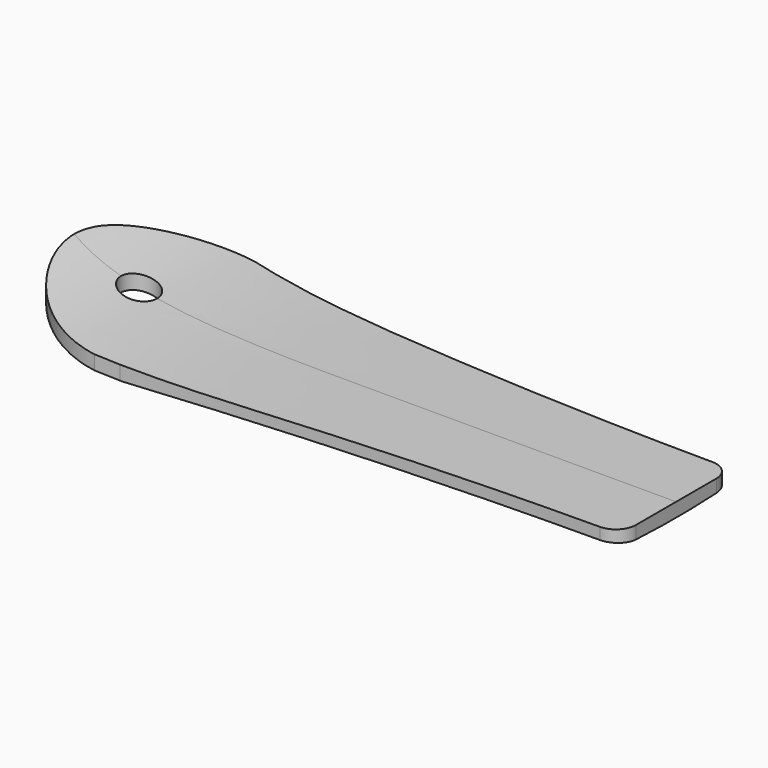
from build123d import *

# Parameters (mm, degrees)
F2_DEPTH = 50
F0_R     = 9
F3_DEPTH = 41
F5_DEPTH = 150


# Not quite as in the source:
# - the dataset's text gives a spline's control points without its knots; the knots are read off the source's solid


with BuildPart() as f2:
    # F1 (on Front) → F2 (new body, symmetric)
    with BuildSketch(Plane.XZ):
        with BuildLine():
            ThreePointArc((-149.9588993892, 26.9134754342), (-154.8613095864, 26.2305586605), (-154.1783928127, 21.3281484633))
            add(Edge.make_bspline(
                [(-154.1783928127, 21.3281484633), (-125.9464059615, 0), (-3.9595449586, 0), (130.4603123693, 0), (151.5675187111, 0)],
                knots=[0, 0, 0, 0, 0.5033195654, 1, 1, 1, 1], degree=3))
            ThreePointArc((151.5675187111, 0), (155.0675187869, 3.5000000758), (151.5675187111, 7.0000001516))
            add(Edge.make_bspline(
                [(-149.9588993892, 26.9134754342), (-148.4478574546, 25.7719430693), (-145.1555512603, 23.5934371829), (-137.5039021405, 19.6641031988), (-126.0184700843, 15.5798750303), (-109.5578013858, 11.9753296087), (-90.8479253185, 9.5246754809), (-70.2937339258, 8.030291433), (-48.2800158692, 7.2686571064), (-29.0264464578, 7.0487772943), (-13.2581336189, 7.0012099028), (-1.291744917, 6.9996863373), (10.7653391732, 7.0000823662), (26.8484793874, 6.9999526881), (46.7909432723, 7.0000162503), (69.87873725, 6.9999959326), (98.7623960141, 7.0000025942), (129.847702251, 6.9999992634), (146.255449604, 7.0000001516), (151.5675187111, 7.0000001516)],
                knots=[0, 0, 0, 0, 0.03125, 0.0625, 0.125, 0.1875, 0.25, 0.3125, 0.375, 0.4375, 0.46875, 0.5, 0.53125, 0.5625, 0.625, 0.6875, 0.75, 0.875, 1, 1, 1, 1], degree=3))
        make_face()
    extrude(amount=F2_DEPTH, both=True)

    # F0 (on Top) → F3 (intersect)
    with BuildSketch(Plane.XY):
        with BuildLine():
            ThreePointArc((-150, 0), (-135.3553390593, -35.3553390593), (-100, -50))
            ThreePointArc((-100, -50), (-94.2011170994, -49.3098342645), (-88.4003291499, -48.635867795))
            ThreePointArc((-88.4003291499, -48.635867795), (-60.7572711034, -30.9839995602), (-50, 0))
            ThreePointArc((-50, 0), (-60.7572711034, 30.9839995602), (-88.4003291499, 48.635867795))
            ThreePointArc((-88.4003291499, 48.635867795), (-94.2011170994, 49.3098342645), (-100, 50))
            ThreePointArc((-100, 50), (-135.3553390593, 35.3553390593), (-150, 0))
        make_face()
        with Locations((-117.6522374153, 0)):
            Circle(F0_R, mode=Mode.SUBTRACT)
        with BuildLine():
            ThreePointArc((140.0476001587, -35.0236869248), (147.0878770301, -32.0780187539), (150, -25.0238002141))
            Line((150, -25.0238002141), (150, 0))
            Line((150, 0), (150, 25.0238002141))
            ThreePointArc((150, 25.0238002141), (147.0878770301, 32.0780187539), (140.0476001587, 35.0236869248))
            ThreePointArc((140.0476001587, 35.0236869248), (25.6372549098, 38.7018244409), (-88.4003291499, 48.635867795))
            ThreePointArc((-88.4003291499, 48.635867795), (-60.7572711034, 30.9839995602), (-50, 0))
            ThreePointArc((-50, 0), (-60.7572711034, -30.9839995602), (-88.4003291499, -48.635867795))
            ThreePointArc((-88.4003291499, -48.635867795), (25.6372549098, -38.7018244409), (140.0476001587, -35.0236869248))
        make_face()
    extrude(amount=F3_DEPTH, mode=Mode.INTERSECT)

    # F4 (on Right) → F5 (intersect, symmetric)
    with BuildSketch(Plane.YZ):
        with BuildLine():
            Line((-52.1002963765, 32.8564588929), (-55.3800071338, 3.0362728213))
            ThreePointArc((-55.3800071338, 3.0362728213), (0, 0), (55.3800071338, 3.0362728213))
            Line((55.3800071338, 3.0362728213), (52.1002963765, 32.8564588929))
            ThreePointArc((52.1002963765, 32.8564588929), (0, 30), (-52.1002963765, 32.8564588929))
        make_face()
    extrude(amount=F5_DEPTH, both=True, mode=Mode.INTERSECT)


solid = f2.part
